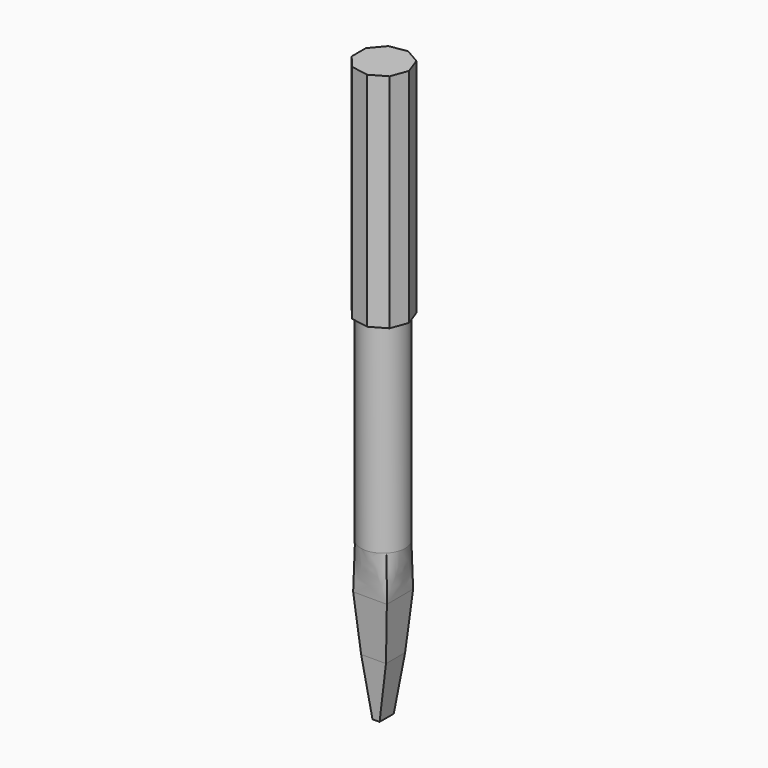
from build123d import *

# Parameters (mm, degrees)
F1_DEPTH = 50
F3_R     = 10
F4_R     = 10
F7_W     = 15.1952523738
F7_H     = 14.7997830063
F10_W    = 11.1952523738
F10_H    = 10.7997830063
F13_W    = 3.1952523738
F13_H    = 8


# Not quite as in the source:
# - the arcs of a loft's sections are written as splines that run evenly, so that the points pair up as in the source's solid


with BuildPart() as f1:
    # F0 (on Top) → F1 (new body, symmetric)
    with BuildSketch(Plane.XY):
        Polygon((-10.9899096778, 4), (-10.9899096778, -4), (-5.8476088003, -10.128355545), (2.0308532238, -11.5175409663), (8.959056454, -7.5175409663), (11.6952176007, 0), (8.959056454, 7.5175409663), (2.0308532238, 11.5175409663), (-5.8476088003, 10.128355545), align=None)
    extrude(amount=F1_DEPTH, both=True)


with BuildPart() as f5:
    # F3 (on offset) → F5 section 0
    with BuildSketch(Plane(origin=(0, 0, -140), x_dir=(1, 0, 0), z_dir=(0, 0, -1))):
        Circle(F3_R)
    # F4 (on face) → F5 section 1
    with BuildSketch(Plane(origin=(0, 0, -50), x_dir=(1, 0, 0), z_dir=(0, 0, -1))):
        Circle(F4_R)
    loft()


with BuildPart() as f8:
    # F3 (on offset) → F8 section 0
    with BuildSketch(Plane(origin=(0, 0, -140), x_dir=(1, 0, 0), z_dir=(0, 0, -1))):
        with BuildLine():
            add(Edge.make_bspline(
                [(7.163673657, 6.977232957), (6.2503559987, 7.9149556459), (5.1509464413, 8.6707106828), (2.7456535845, 9.704373209), (1.4407166651, 9.9818739963), (-1.1770496985, 10.0163879215), (-2.4888491633, 9.7733874797), (-4.9205578349, 8.8034983717), (-6.0395102681, 8.0769913154), (-6.977232957, 7.163673657)],
                knots=[0, 0, 0, 0, 0.25, 0.25, 0.5, 0.5, 0.75, 0.75, 1, 1, 1, 1], degree=3))
            add(Edge.make_bspline(
                [(-6.977232957, 7.163673657), (-7.9149556459, 6.2503559987), (-8.6707106828, 5.1509464413), (-9.704373209, 2.7456535845), (-9.9818739963, 1.4407166651), (-10.0163879215, -1.1770496985), (-9.7733874797, -2.4888491633), (-8.8034983717, -4.9205578349), (-8.0769913154, -6.0395102681), (-7.163673657, -6.977232957)],
                knots=[0, 0, 0, 0, 0.25, 0.25, 0.5, 0.5, 0.75, 0.75, 1, 1, 1, 1], degree=3))
            add(Edge.make_bspline(
                [(-7.163673657, -6.977232957), (-6.2503559987, -7.9149556459), (-5.1509464413, -8.6707106828), (-2.7456535845, -9.704373209), (-1.4407166651, -9.9818739963), (1.1770496985, -10.0163879215), (2.4888491633, -9.7733874797), (4.9205578349, -8.8034983717), (6.0395102681, -8.0769913154), (6.977232957, -7.163673657)],
                knots=[0, 0, 0, 0, 0.25, 0.25, 0.5, 0.5, 0.75, 0.75, 1, 1, 1, 1], degree=3))
            add(Edge.make_bspline(
                [(6.977232957, -7.163673657), (7.9149556459, -6.2503559987), (8.6707106828, -5.1509464413), (9.704373209, -2.7456535845), (9.9818739963, -1.4407166651), (10.0163879215, 1.1770496985), (9.7733874797, 2.4888491633), (8.8034983717, 4.9205578349), (8.0769913154, 6.0395102681), (7.163673657, 6.977232957)],
                knots=[0, 0, 0, 0, 0.25, 0.25, 0.5, 0.5, 0.75, 0.75, 1, 1, 1, 1], degree=3))
        make_face()
    # F7 (on offset) → F8 section 1
    with BuildSketch(Plane(origin=(0, 0, -160), x_dir=(1, 0, 0), z_dir=(0, 0, -1))):
        Rectangle(F7_W, F7_H)
    loft(ruled=True)

    # F7 (on offset) → F11 section 0
    with BuildSketch(Plane(origin=(0, 0, -160), x_dir=(1, 0, 0), z_dir=(0, 0, -1))):
        Rectangle(F7_W, F7_H)
    # F10 (on offset) → F11 section 1
    with BuildSketch(Plane(origin=(0, 0, -185), x_dir=(1, 0, 0), z_dir=(0, 0, -1))):
        Rectangle(F10_W, F10_H)
    loft()


with BuildPart() as f14:
    # F10 (on offset) → F14 section 0
    with BuildSketch(Plane(origin=(0, 0, -185), x_dir=(1, 0, 0), z_dir=(0, 0, -1))):
        Rectangle(F10_W, F10_H)
    # F13 (on offset) → F14 section 1
    with BuildSketch(Plane(origin=(0, 0, -210), x_dir=(1, 0, 0), z_dir=(0, 0, -1))):
        Rectangle(F13_W, F13_H)
    loft()


solid = Compound([f1.part, f5.part, f8.part, f14.part])
